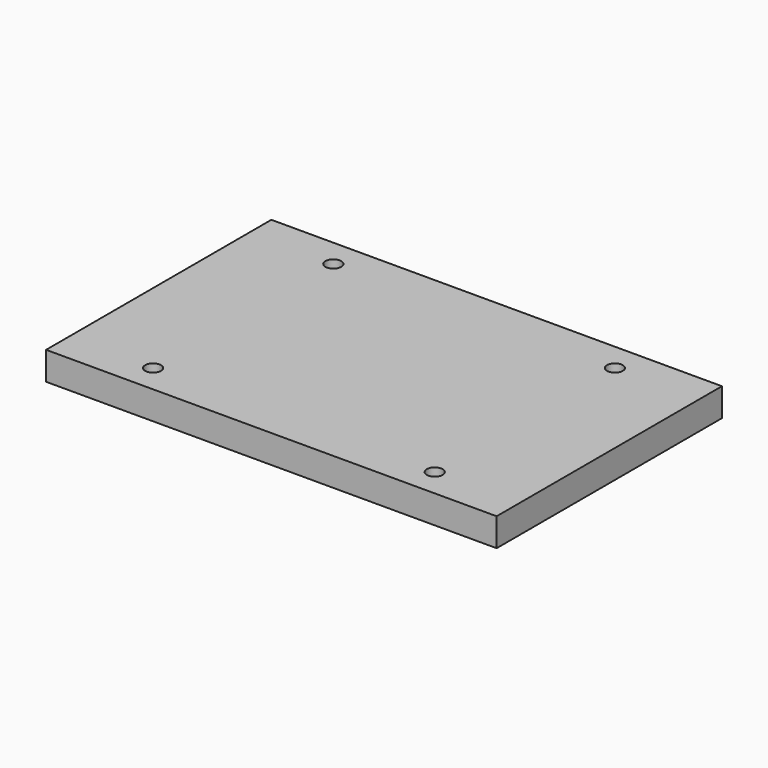
from build123d import *

# Parameters (mm, degrees)
F0_W     = 101.6
F0_H     = 63.5
F0_R     = 1.778
F1_DEPTH = 6.35


# Not quite as in the source:
# - a length typed as a fraction of an inch, garbled in the dataset ("3 / 203.2 mm" for 3/8 in), is restored


with BuildPart() as f1:
    # F0 (on Top) → F1 (new body)
    with BuildSketch(Plane.XY):
        with Locations((50.8, 31.75)):
            Rectangle(F0_W, F0_H)
        with Locations((19.05, 6.35)):
            Circle(F0_R, mode=Mode.SUBTRACT)
        with Locations((82.55, 6.35)):
            Circle(F0_R, mode=Mode.SUBTRACT)
        with Locations((19.05, 57.15)):
            Circle(F0_R, mode=Mode.SUBTRACT)
        with Locations((82.55, 57.15)):
            Circle(F0_R, mode=Mode.SUBTRACT)
    extrude(amount=F1_DEPTH)


solid = f1.part
